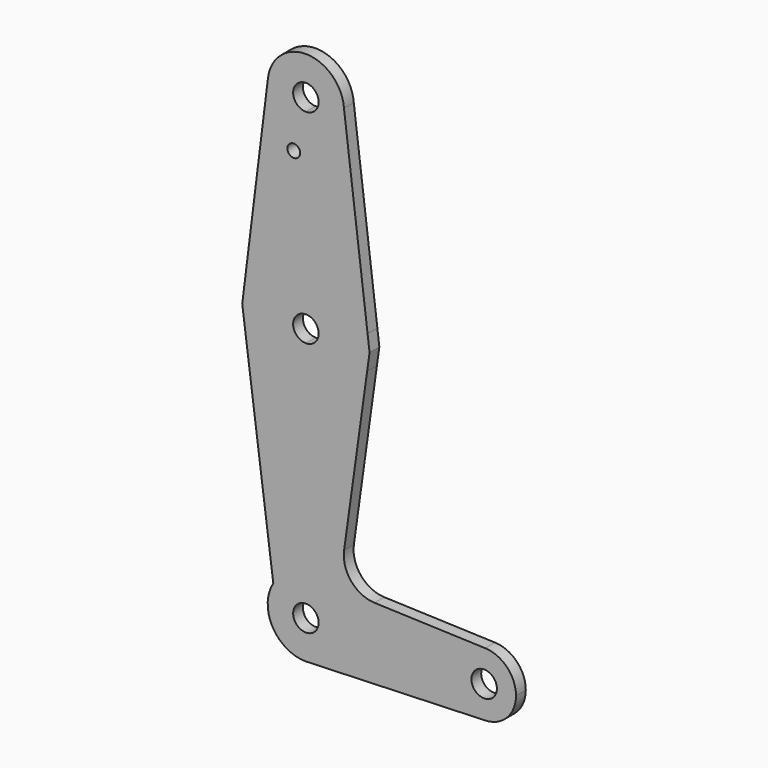
from build123d import *

# Parameters (mm, degrees)
F0_R     = 1.5875
F1_DEPTH = 3.048


with BuildPart() as f1:
    # F0 (on Front) → F1 (new body)
    with BuildSketch(Plane.XZ):
        with BuildLine():
            ThreePointArc((0, 3.175), (2.2450640303, 2.2450640303), (3.175, 0))
            Line((3.175, 0), (9.525, 0))
            ThreePointArc((9.525, 0), (6.7351920908, 6.7351920908), (0, 9.525))
            Line((0, 9.525), (0, 3.175))
        make_face()
        with BuildLine():
            Line((9.525, 0), (3.175, 0))
            ThreePointArc((3.175, 0), (-2.2450640303, -2.2450640303), (0, 3.175))
            Line((0, 3.175), (0, 9.525))
            ThreePointArc((0, 9.525), (-4.6545218696, 8.3102978987), (-8.1218820604, 4.9760081187))
            ThreePointArc((-8.1218820604, 4.9760081187), (-8.3102978987, -4.6545218696), (0, -9.525))
            Line((0, -9.525), (0.6773435479, -9.500885786))
            ThreePointArc((0.6773435479, -9.500885786), (6.9705567315, -6.4912990883), (9.525, 0))
        make_face()
        with BuildLine():
            ThreePointArc((0, 9.525), (6.7351920908, 6.7351920908), (9.525, 0))
            Line((9.525, 0), (36.5125, 0))
            ThreePointArc((36.5125, 0), (38.9380895153, 5.7116327839), (44.7324052746, 7.9324746146))
            Line((44.7324052746, 7.9324746146), (17.1156877493, 8.9156617124))
            ThreePointArc((17.1156877493, 8.9156617124), (11.3089068229, 11.7498608175), (9.5247208389, 17.9601804284))
            Line((9.5247208389, 17.9601804284), (15.2838268526, 59.2082806579))
            ThreePointArc((15.2838268526, 59.2082806579), (9.588626561, 50.8480047791), (0, 47.6250000001))
            Line((0, 47.6250000001), (0, 9.525))
        make_face()
        with BuildLine():
            Line((36.5125, 0), (9.525, 0))
            ThreePointArc((9.525, 0), (6.9705567315, -6.4912990883), (0.6773435479, -9.500885786))
            Line((0.6773435479, -9.500885786), (44.7324052746, -7.9324746146))
            ThreePointArc((44.7324052746, -7.9324746146), (38.9380895153, -5.7116327839), (36.5125, 0))
        make_face()
        with BuildLine():
            ThreePointArc((-8.1218820604, 4.9760081187), (-4.6545218696, 8.3102978987), (0, 9.525))
            Line((0, 9.525), (0, 47.6250000001))
            ThreePointArc((0, 47.6250000001), (-9.5462552297, 50.8159346111), (-15.2548293812, 59.106002992))
            Line((-15.2548293812, 59.106002992), (-8.1218820604, 4.9760081187))
        make_face()
        with BuildLine():
            ThreePointArc((44.7324052746, 7.9324746146), (38.9380895153, 5.7116327839), (36.5125, 0))
            ThreePointArc((36.5125, 0), (38.9380895153, -5.7116327839), (44.7324052746, -7.9324746146))
            ThreePointArc((44.7324052746, -7.9324746146), (50.1616327839, -5.5119104847), (52.3875, 0))
            ThreePointArc((52.3875, 0), (50.1616327839, 5.5119104847), (44.7324052746, 7.9324746146))
        make_face()
        with BuildLine():
            ThreePointArc((47.625, 0), (44.45, -3.175), (41.275, 0))
            ThreePointArc((41.275, 0), (44.45, 3.175), (47.625, 0))
        make_face(mode=Mode.SUBTRACT)
        with BuildLine():
            Line((0, 60.3250000003), (0, 47.6250000001))
            ThreePointArc((0, 47.6250000001), (9.588626561, 50.8480047791), (15.2838268526, 59.2082806579))
            Line((15.2838268526, 59.2082806579), (15.8748454422, 63.4412977202))
            Line((15.8748454422, 63.4412977202), (15.3823268829, 67.4240576925))
            ThreePointArc((15.3823268829, 67.4240576925), (9.7396130333, 76.0361344305), (0, 79.3749999999))
            Line((0, 79.3749999999), (0, 66.6749999997))
            ThreePointArc((0, 66.6749999997), (2.2450342786, 65.7450477585), (3.1749539767, 63.5))
            ThreePointArc((3.1749539767, 63.5), (2.2450342786, 61.2549522415), (0, 60.3250000003))
        make_face()
        with BuildLine():
            ThreePointArc((-15.2548293812, 59.106002992), (-9.5462552297, 50.8159346111), (0, 47.6250000001))
            Line((0, 47.6250000001), (0, 60.3250000003))
            ThreePointArc((0, 60.3250000003), (-3.1750460233, 63.5), (0, 66.6749999997))
            Line((0, 66.6749999997), (0, 79.3749999999))
            ThreePointArc((0, 79.3749999999), (-9.870803232, 75.9331724482), (-15.4614519338, 67.1000767036))
            Line((-15.4614519338, 67.1000767036), (-15.872355841, 63.7922431396))
            Line((-15.872355841, 63.7922431396), (-15.2548293812, 59.106002992))
        make_face()
        with BuildLine():
            Line((-9.452349728, 115.474184662), (-15.4614519338, 67.1000767036))
            ThreePointArc((-15.4614519338, 67.1000767036), (-9.870803232, 75.9331724482), (0, 79.3749999999))
            Line((0, 79.3749999999), (0, 104.775))
            ThreePointArc((0, 104.775), (-7.1382677838, 107.9935938882), (-9.452349728, 115.474184662))
        make_face()
        with Locations((-3.0307907145, 101.5941351652)):
            Circle(F0_R, mode=Mode.SUBTRACT)
        with BuildLine():
            ThreePointArc((0, 79.3749999999), (9.7396130333, 76.0361344305), (15.3823268829, 67.4240576925))
            Line((15.3823268829, 67.4240576925), (9.4996558287, 114.9943803979))
            ThreePointArc((9.4996558287, 114.9943803979), (9.5186618484, 114.647421381), (9.525, 114.3))
            ThreePointArc((9.525, 114.3), (6.7351920908, 107.5648079092), (0, 104.775))
            Line((0, 104.775), (0, 79.3749999999))
        make_face()
        with BuildLine():
            ThreePointArc((9.4996558287, 114.9943803979), (0.2410653433, 123.8219489864), (-9.452349728, 115.474184662))
            ThreePointArc((-9.452349728, 115.474184662), (-7.1382677838, 107.9935938882), (0, 104.775))
            ThreePointArc((0, 104.775), (6.7351920908, 107.5648079092), (9.525, 114.3))
            ThreePointArc((9.525, 114.3), (9.5186618484, 114.647421381), (9.4996558287, 114.9943803979))
        make_face()
        with BuildLine():
            ThreePointArc((3.175, 114.3), (2.2450640303, 112.0549359697), (0, 111.125))
            ThreePointArc((0, 111.125), (-2.2450640303, 116.5450640303), (3.175, 114.3))
        make_face(mode=Mode.SUBTRACT)
    extrude(amount=F1_DEPTH)


solid = f1.part
